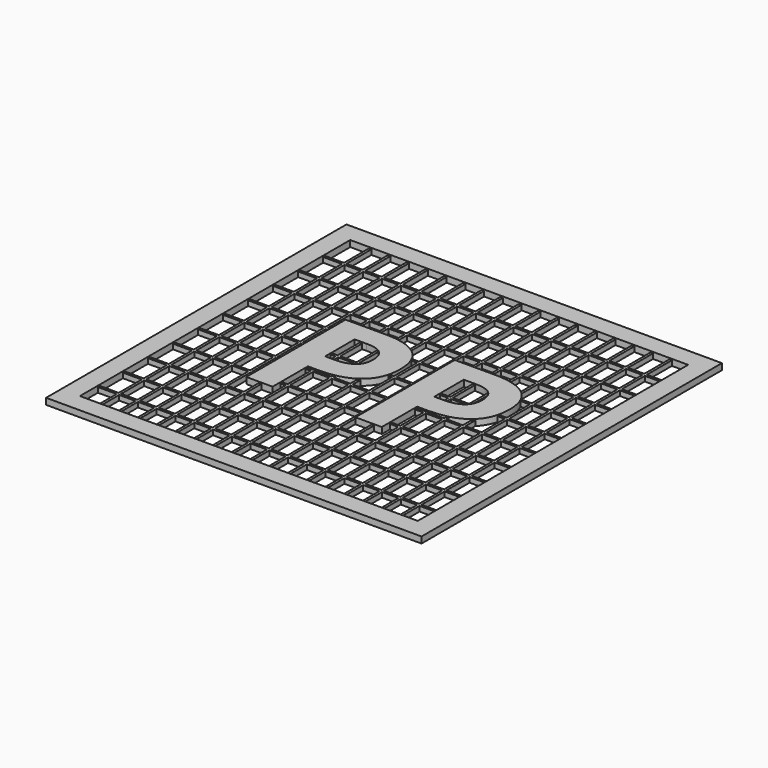
from build123d import *

# Parameters (mm, degrees)
F0_W         = 120
F0_H         = 120
F0_W_2       = 108
F0_H_2       = 108
F1_DEPTH     = 2
F2_W         = 118
F2_H         = 0.8
F3_DEPTH     = 1.6
F4_W         = 0.8
F4_H         = 115
F5_DEPTH     = 1.6
F6_TEXT_SIZE = 55.5555555556
F7_DEPTH     = 2


# Not quite as in the source:
# - Text() gives the source's letters only with a copy of the font that has no kerning and outlines rounded to 1/6400 em; it was checked with that copy


with BuildPart() as f1:
    # F0 (on Top) → F1 (new body)
    with BuildSketch(Plane.XY):
        with Locations((-1, 0)):
            Rectangle(F0_W, F0_H)
        with Locations((-1, 0)):
            Rectangle(F0_W_2, F0_H_2, mode=Mode.SUBTRACT)
    extrude(amount=F1_DEPTH)

    # F2 (on Top) → F3 (join)
    with BuildSketch(Plane.XY):
        with Locations((-1, 43.6)):
            Rectangle(F2_W, F2_H)
        with Locations((-0.9925439034, 33.6000027797)):
            Rectangle(F2_W, F2_H)
        with Locations((-0.9850878068, 23.6000055593)):
            Rectangle(F2_W, F2_H)
        with Locations((-0.9776317101, 13.600008339)):
            Rectangle(F2_W, F2_H)
        with Locations((-0.9701756135, 3.6000111187)):
            Rectangle(F2_W, F2_H)
        with Locations((-0.9627195169, -6.3999861017)):
            Rectangle(F2_W, F2_H)
        with Locations((-0.9552634203, -16.399983322)):
            Rectangle(F2_W, F2_H)
        with Locations((-0.9478073237, -26.3999805423)):
            Rectangle(F2_W, F2_H)
        with Locations((-0.940351227, -36.3999777626)):
            Rectangle(F2_W, F2_H)
        with Locations((-0.9328951304, -46.399974983)):
            Rectangle(F2_W, F2_H)
    extrude(amount=F3_DEPTH)

    # F4 (on Top) → F5 (join)
    with BuildSketch(Plane.XY):
        with Locations((-48.6, -0.1633819193)):
            Rectangle(F4_W, F4_H)
        with Locations((-42.6, -0.1633819193)):
            Rectangle(F4_W, F4_H)
        with Locations((-36.6, -0.1633819193)):
            Rectangle(F4_W, F4_H)
        with Locations((-30.6, -0.1633819193)):
            Rectangle(F4_W, F4_H)
        with Locations((-24.6, -0.1633819193)):
            Rectangle(F4_W, F4_H)
        with Locations((-18.6, -0.1633819193)):
            Rectangle(F4_W, F4_H)
        with Locations((-12.6, -0.1633819193)):
            Rectangle(F4_W, F4_H)
        with Locations((-6.6, -0.1633819193)):
            Rectangle(F4_W, F4_H)
        with Locations((-0.6, -0.1633819193)):
            Rectangle(F4_W, F4_H)
        with Locations((5.4, -0.1633819193)):
            Rectangle(F4_W, F4_H)
        with Locations((11.4, -0.1633819193)):
            Rectangle(F4_W, F4_H)
        with Locations((17.4, -0.1633819193)):
            Rectangle(F4_W, F4_H)
        with Locations((23.4, -0.1633819193)):
            Rectangle(F4_W, F4_H)
        with Locations((29.4, -0.1633819193)):
            Rectangle(F4_W, F4_H)
        with Locations((35.4, -0.1633819193)):
            Rectangle(F4_W, F4_H)
        with Locations((41.4, -0.1633819193)):
            Rectangle(F4_W, F4_H)
        with Locations((47.4, -0.1633819193)):
            Rectangle(F4_W, F4_H)
    extrude(amount=F5_DEPTH)

    # F6 (on Top) → F7 (join)
    with BuildSketch(Plane.XY):
        with Locations((-34, -20)):
            Text('PP', F6_TEXT_SIZE, font='Open Sans', font_style=FontStyle.BOLD, text_align=(TextAlign.LEFT, TextAlign.BOTTOM))
    extrude(amount=F7_DEPTH)


solid = f1.part
